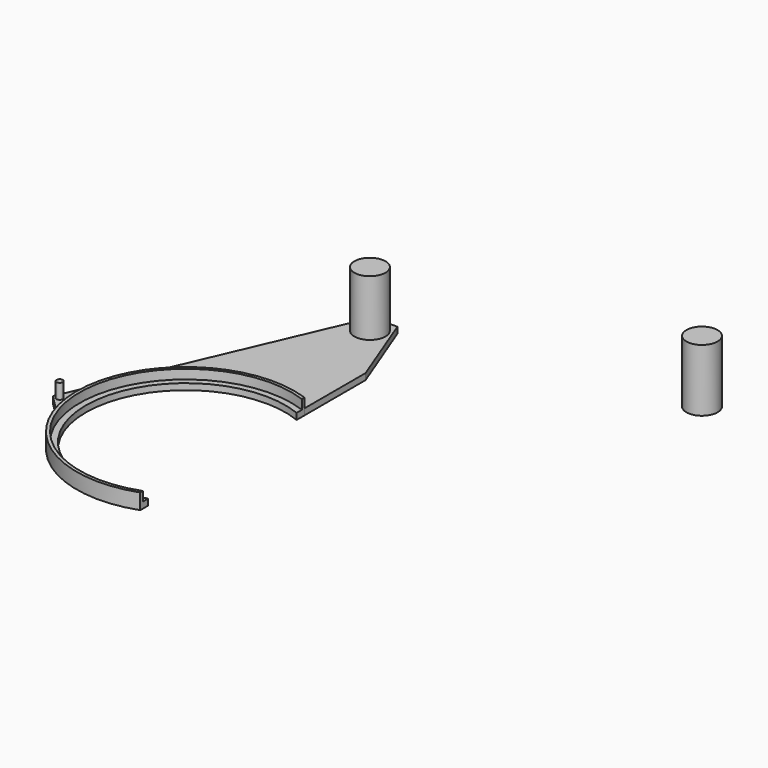
from build123d import *

# Parameters (mm, degrees)
F1_DEPTH = 10
F2_DEPTH = 25
F0_R     = 25
F3_DEPTH = 100
F0_R_2   = 5
F4_DEPTH = 10
F5_DEPTH = 34
F6_DEPTH = 100


# Not quite as in the source:
# - a feature names something its author has since deleted; it is built from what else it names


with BuildPart() as f1:
    # F0 (on Top) → F1 (new body)
    with BuildSketch(Plane.XY):
        with BuildLine():
            Line((620.0774312019, 723.5964589473), (620.0774312019, 734.3029628668))
            ThreePointArc((620.0774312019, 734.3029628668), (391.1634666106, 574.8377792808), (620.0774312019, 415.3725956948))
            Line((620.0774312019, 415.3725956948), (620.0774312019, 426.0790996143))
            ThreePointArc((620.0774312019, 426.0790996143), (401.1634666106, 574.8377792808), (620.0774312019, 723.5964589473))
        make_face()
    extrude(amount=F1_DEPTH)

    # F0 (on Top) → F2 (join)
    with BuildSketch(Plane.XY):
        with BuildLine():
            Line((620.0774312019, 734.3029628668), (620.0774312019, 739.6229265973))
            ThreePointArc((620.0774312019, 739.6229265973), (460.3789038132, 717.9023517708), (386.1634666106, 574.8377792808))
            ThreePointArc((386.1634666106, 574.8377792808), (387.6389733709, 552.1606929179), (392.0406122781, 529.8660087749))
            ThreePointArc((392.0406122781, 529.8660087749), (479.7674522107, 419.9194497009), (620.0774312019, 410.0526319643))
            Line((620.0774312019, 410.0526319643), (620.0774312019, 415.3725956948))
            ThreePointArc((620.0774312019, 415.3725956948), (391.1634666106, 574.8377792808), (620.0774312019, 734.3029628668))
        make_face()
    extrude(amount=F2_DEPTH)


with BuildPart() as f3:
    # F0 (on Top) → F3 (new body)
    with BuildSketch(Plane.XY):
        with Locations((552.6312583531, 954.8377792808)):
            Circle(F0_R)
    extrude(amount=F3_DEPTH)


with BuildPart() as f4:
    # F0 (on Top) → F4 (new body)
    with BuildSketch(Plane.XY):
        with BuildLine():
            ThreePointArc((392.0406122781, 529.8660087749), (387.6389733709, 552.1606929179), (386.1634666106, 574.8377792808))
            Line((386.1634666106, 574.8377792808), (386.1634666106, 644.8377792808))
            Line((386.1634666106, 644.8377792808), (353.2142043114, 568.3516860008))
            Line((353.2142043114, 568.3516860008), (392.0406122781, 529.8660087749))
        make_face()
        with Locations((363.1972372532, 569.6715116501)):
            Circle(F0_R_2, mode=Mode.SUBTRACT)
        with BuildLine():
            ThreePointArc((386.1634666106, 574.8377792808), (460.3789038132, 717.9023517708), (620.0774312019, 739.6229265973))
            Line((620.0774312019, 739.6229265973), (620.0774312019, 861.8070483208))
            Line((620.0774312019, 861.8070483208), (572.6312583531, 984.8377792808))
            Line((572.6312583531, 984.8377792808), (532.6312583531, 984.8377792808))
            Line((532.6312583531, 984.8377792808), (386.1634666106, 644.8377792808))
            Line((386.1634666106, 644.8377792808), (386.1634666106, 574.8377792808))
        make_face()
        with Locations((552.6312583531, 954.8377792808)):
            Circle(F0_R, mode=Mode.SUBTRACT)
    extrude(amount=F4_DEPTH)

    # F0 (on Top) → F5 (join)
    with BuildSketch(Plane.XY):
        with Locations((363.1972372532, 569.6715116501)):
            Circle(F0_R_2)
    extrude(amount=F5_DEPTH)


with BuildPart() as f6:
    # F0 (on Top) → F6 (new body)
    with BuildSketch(Plane.XY):
        with Locations((993.8411712646, 1069.0063238144)):
            Circle(F0_R)
    extrude(amount=F6_DEPTH)


solid = Compound([f1.part, f3.part, f4.part, f6.part])
